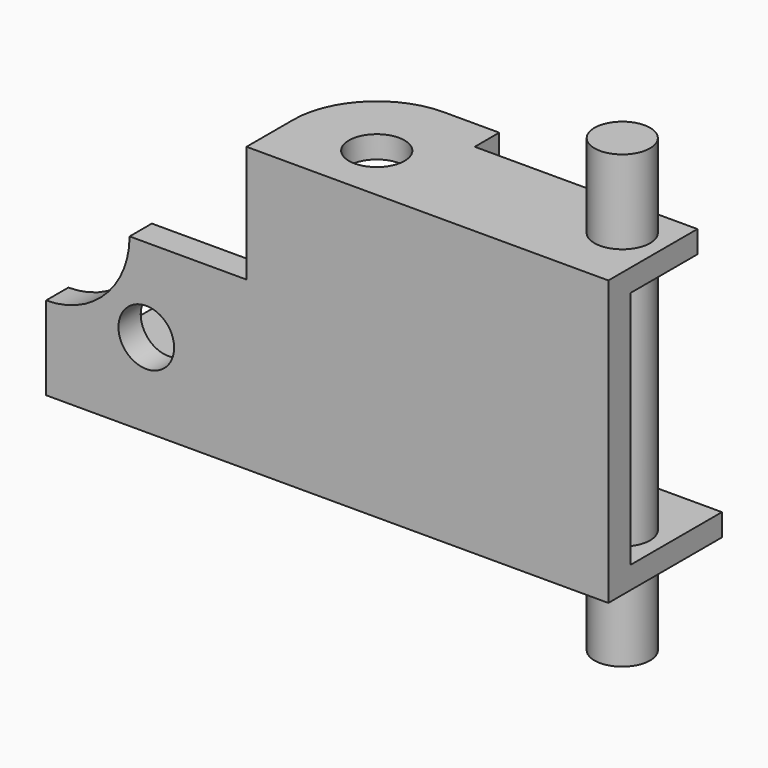
from build123d import *

# Parameters (mm, degrees)
F1_DEPTH  = 10
F2_R      = 29.99999
F4_D      = 20
F5_W      = 202
F5_H      = 41
F6_DEPTH  = 8
F8_D      = 20
F10_DEPTH = 8
F11_R     = 30
F13_D     = 20
F14_D     = 20
F15_R     = 9.9871589088
F16_DEPTH = 30
F17_R     = 9.9871589088
F18_DEPTH = 132


# Not quite as in the source:
# - a fillet or chamfer is up to 0.001 mm smaller than in the source, because OpenCascade refuses the exact size


with BuildPart() as f1:
    # F0 (on Front) → F1 (new body)
    with BuildSketch(Plane.XZ):
        Polygon((-202, 0), (0, 0), (0, 102), (-130, 102), (-130, 60), (-172, 60), (-172, 30), (-202, 30), align=None)
    extrude(amount=F1_DEPTH)

    # F2 (radius 30 in the source; OpenCascade refuses exactly that, so slightly less here)
    f2_edges = [f1.edges().sort_by_distance(p)[0] for p in [
        (-172, -5, 30),
    ]]
    fillet(f2_edges, radius=F2_R)

    # F4 (through all)
    with Locations(Plane.XZ.offset(10)):
        with Locations((-166, 30)):
            Hole(F4_D / 2)

    # F5 (on Top) → F6 (join)
    with BuildSketch(Plane.XY):
        with Locations((-101, 20.5)):
            Rectangle(F5_W, F5_H)
    extrude(amount=F6_DEPTH)

    # F8 (through all)
    with Locations(Plane(origin=(0, 0, 0), x_dir=(1, 0, 0), z_dir=(0, 0, -1))):
        with Locations((-15, -15)):
            Hole(F8_D / 2)

    # F9 (on face) → F10 (join)
    with BuildSketch(Plane.XY.offset(102)):
        Polygon((-130, 0), (0, 0), (0, 30), (-80, 30), (-80, 41), (-130, 41), align=None)
    extrude(amount=-F10_DEPTH)

    # F11
    f11_edges = [f1.edges().sort_by_distance(p)[0] for p in [
        (-130, 41, 98),
    ]]
    fillet(f11_edges, radius=F11_R)

    # F13 (through all)
    with Locations(Plane.XY.offset(102)):
        with Locations((-100, 11)):
            Hole(F13_D / 2)

    # F14 (through all)
    with Locations(Plane.XY.offset(102)):
        with Locations((-15, 15)):
            Hole(F14_D / 2)


with BuildPart() as f16:
    # F15 (on face) → F16 (new body)
    with BuildSketch(Plane.XY.offset(102)):
        with Locations((-15, 15)):
            Circle(F15_R)
    extrude(amount=F16_DEPTH)

    # F17 (on face) → F18 (join)
    with BuildSketch(Plane(origin=(0, 0, 102), x_dir=(1, 0, 0), z_dir=(0, 0, -1))):
        with Locations((-15, -15)):
            Circle(F17_R)
    extrude(amount=F18_DEPTH)


solid = Compound([f1.part, f16.part])
